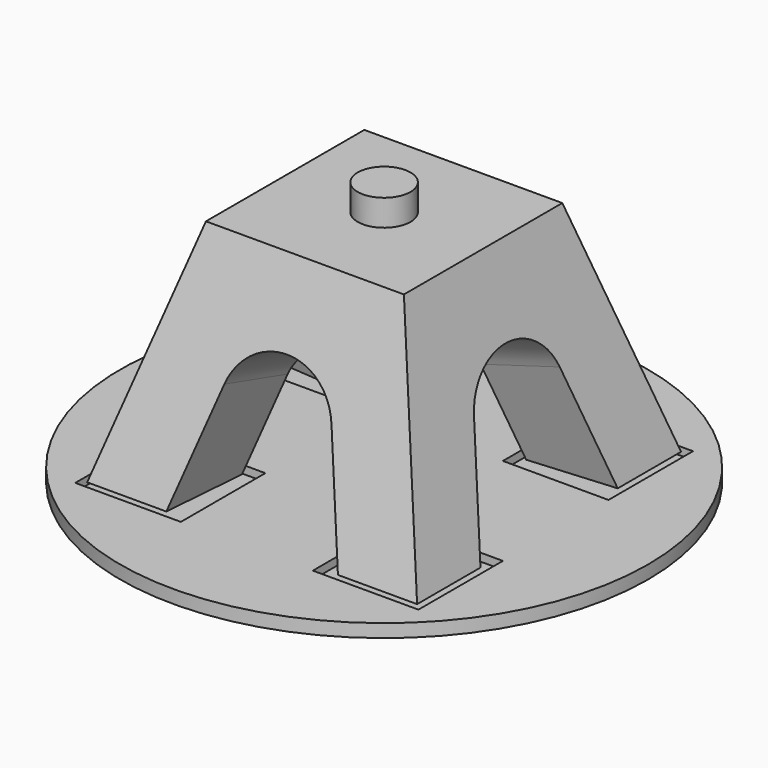
from build123d import *

# Parameters (mm, degrees)
F0_R      = 25.4
F1_DEPTH  = 1.27
F2_W      = 31.75
F2_H      = 31.75
F4_W      = 19.05
F4_H      = 19.05
F10_DEPTH = 74.422
F11_DEPTH = 67.7926
F12_DEPTH = 25.4
F13_DEPTH = 25.4
F14_W     = 10.16
F14_H     = 10.16
F15_DEPTH = 0.762
F16_R     = 2.54
F17_DEPTH = 2.54
F18_R     = 3.429
F19_DEPTH = 25.4


with BuildPart() as f1:
    # F0 (on Top) → F1 (new body)
    with BuildSketch(Plane.XY):
        Circle(F0_R)
    extrude(amount=-F1_DEPTH)

    # F14 (on face) → F15 (cut)
    with BuildSketch(Plane.XY):
        with Locations((11.43, 11.43)):
            Rectangle(F14_W, F14_H)
        with Locations((11.43, -11.43)):
            Rectangle(F14_W, F14_H)
        with Locations((-11.43, 11.43)):
            Rectangle(F14_W, F14_H)
        with Locations((-11.43, -11.43)):
            Rectangle(F14_W, F14_H)
    extrude(amount=-F15_DEPTH, mode=Mode.SUBTRACT)

    # F18 (on face) → F19 (cut)
    with BuildSketch(Plane.XY):
        Circle(F18_R)
    extrude(amount=-F19_DEPTH, mode=Mode.SUBTRACT)


with BuildPart() as f5:
    # F2 (on Top) → F5 section 0
    with BuildSketch(Plane.XY):
        Rectangle(F2_W, F2_H)
    # F4 (on offset) → F5 section 1
    with BuildSketch(Plane.XY.offset(21.59)):
        Rectangle(F4_W, F4_H)
    loft()

    # F9 (on face) → F10 (cut)
    with BuildSketch(Plane(origin=(14.611066879, 0, 4.2973726115), x_dir=(0, 1, 0), z_dir=(0.9593655016, 0, 0.282166324))):
        with BuildLine():
            Line((-8.255, -4.4793903934), (8.255, -4.4793903934))
            Line((8.255, -4.4793903934), (5.1563233946, 6.5023474752))
            ThreePointArc((5.1563233946, 6.5023474752), (0, 10.4050669429), (-5.1563233946, 6.5023474752))
            Line((-5.1563233946, 6.5023474752), (-8.255, -4.4793903934))
        make_face()
    extrude(amount=-F10_DEPTH, mode=Mode.SUBTRACT)

    # F6 (on face) → F11 (cut)
    with BuildSketch(Plane(origin=(0, -14.611066879, 4.2973726115), x_dir=(1, 0, 0), z_dir=(0, -0.9593655016, 0.282166324))):
        with BuildLine():
            Line((-8.255, -4.4793903934), (8.255, -4.4793903934))
            Line((8.255, -4.4793903934), (5.1563233946, 6.5023474752))
            ThreePointArc((5.1563233946, 6.5023474752), (0, 10.4050669429), (-5.1563233946, 6.5023474752))
            Line((-5.1563233946, 6.5023474752), (-8.255, -4.4793903934))
        make_face()
    extrude(amount=-F11_DEPTH, mode=Mode.SUBTRACT)

    # F7 (on face) → F12 (cut)
    with BuildSketch(Plane(origin=(0, 14.611066879, 4.2973726115), x_dir=(-1, 0, 0), z_dir=(0, 0.9593655016, 0.282166324))):
        with BuildLine():
            Line((-8.255, -4.4793903934), (8.255, -4.4793903934))
            Line((8.255, -4.4793903934), (5.1563233946, 6.5023474752))
            ThreePointArc((5.1563233946, 6.5023474752), (0, 10.4050669429), (-5.1563233946, 6.5023474752))
            Line((-5.1563233946, 6.5023474752), (-8.255, -4.4793903934))
        make_face()
    extrude(amount=-F12_DEPTH, mode=Mode.SUBTRACT)

    # F8 (on face) → F13 (cut)
    with BuildSketch(Plane(origin=(-14.611066879, 0, 4.2973726115), x_dir=(0, -1, 0), z_dir=(-0.9593655016, 0, 0.282166324))):
        with BuildLine():
            Line((-5.1563233946, 6.5023474752), (-8.255, -4.4793903934))
            Line((-8.255, -4.4793903934), (8.255, -4.4793903934))
            Line((8.255, -4.4793903934), (5.1563233946, 6.5023474752))
            ThreePointArc((5.1563233946, 6.5023474752), (0, 10.4050669429), (-5.1563233946, 6.5023474752))
        make_face()
    extrude(amount=-F13_DEPTH, mode=Mode.SUBTRACT)

    # F16 (on face) → F17 (join)
    with BuildSketch(Plane.XY.offset(21.59)):
        Circle(F16_R)
    extrude(amount=F17_DEPTH)


solid = Compound([f1.part, f5.part])
